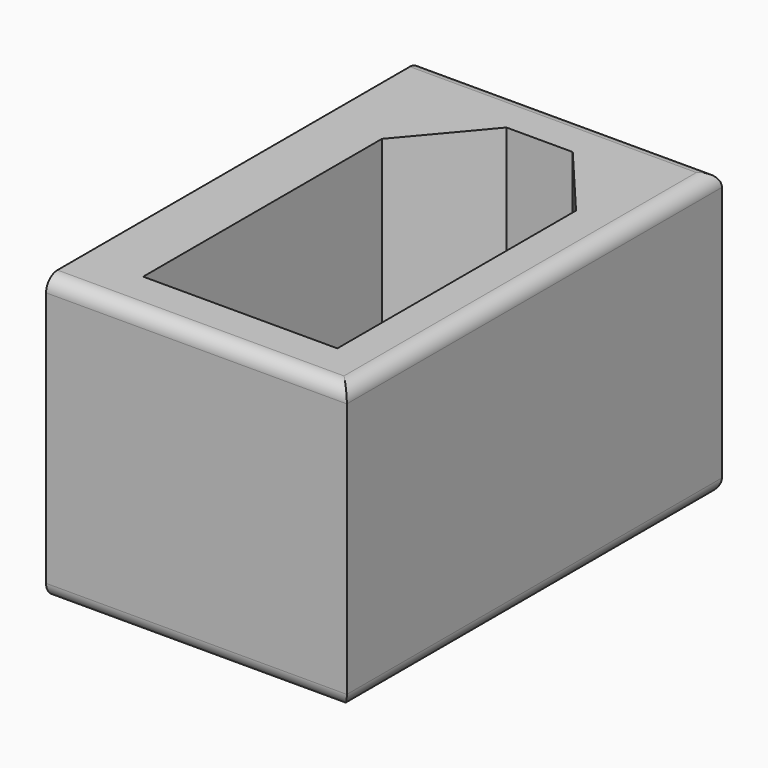
from build123d import *

# Parameters (mm, degrees)
F0_W     = 12.7
F0_H     = 19.8
F1_DEPTH = 12
F0_R     = 2.75
F2_DEPTH = 2
F3_R     = 0.6
F4_R     = 0.6


# Not quite as in the source:
# - a feature names something its author has since deleted; it is built from what else it names


with BuildPart() as f1:
    # F0 (on Top) → F1 (new body)
    with BuildSketch(Plane.XY):
        with Locations((13.45, 9.9)):
            Rectangle(F0_W, F0_H)
        Polygon((17.8, 14.6), (17.8, 2), (9.6, 2), (9.6, 14.6), (12.3, 17.8), (15.1, 17.8), align=None, mode=Mode.SUBTRACT)
    extrude(amount=F1_DEPTH)

    # F0 (on Top) → F2 (join)
    with BuildSketch(Plane.XY):
        Polygon((9.6, 2), (17.8, 2), (17.8, 14.6), (15.1, 17.8), (12.3, 17.8), (9.6, 14.6), align=None)
        with Locations((13.7, 6.1)):
            Circle(F0_R, mode=Mode.SUBTRACT)
        with Locations((13.7, 13.1)):
            Circle(F0_R, mode=Mode.SUBTRACT)
    extrude(amount=F2_DEPTH)

    # F3
    f3_edges = [f1.edges().sort_by_distance(p)[0] for p in [
        (13.45, 0, 12),
        (19.8, 9.9, 12),
        (13.45, 19.8, 12),
    ]]
    fillet(f3_edges, radius=F3_R)

    # F4
    f4_edges = [f1.edges().sort_by_distance(p)[0] for p in [
        (13.45, 0, 0),
        (19.8, 9.9, 0),
        (13.45, 19.8, 0),
    ]]
    fillet(f4_edges, radius=F4_R)


solid = f1.part
